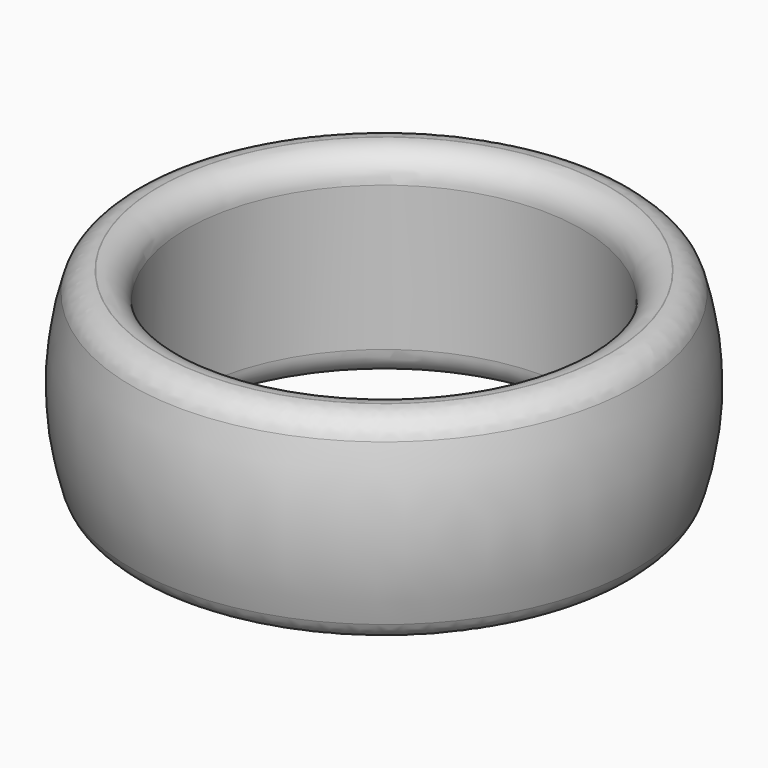
from build123d import *

# Parameters (mm, degrees)
F2_R = 1.3208


with BuildPart() as f1:
    # F0 (on Front) → F1 (revolve)
    with BuildSketch(Plane.XZ):
        with BuildLine():
            Line((9.4, 0), (11.686, 0))
            ThreePointArc((11.686, 0), (12.5745090304, 4.7625), (11.686, 9.525))
            Line((11.686, 9.525), (9.4, 9.525))
            Line((9.4, 9.525), (9.4, 0))
        make_face()
    revolve(axis=Axis((0, 0, 4.7625), (0, 0, -1)))

    # F2
    f2_edges = [f1.edges().sort_by_distance(p)[0] for p in [
        (-11.686, 0, 9.525),
        (-11.686, 0, 0),
        (-9.4, 0, 9.525),
        (-9.4, 0, 0),
    ]]
    fillet(f2_edges, radius=F2_R)


solid = f1.part
